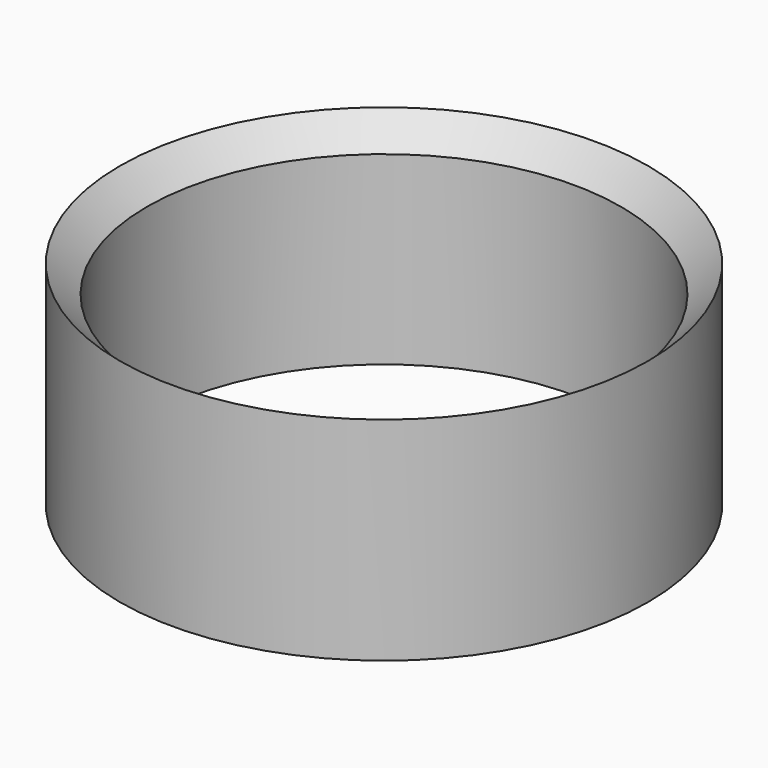
from build123d import *

# Parameters (mm, degrees)
F0_R     = 27.375
F0_R_2   = 24.565
F1_DEPTH = 22.09


# Not quite as in the source:
# - a fillet or chamfer that OpenCascade refuses, or shapes differently, is made with other operations: its cross-section is extruded or revolved along the edge and cut away or added


with BuildPart() as f1:
    # F0 (on Top) → F1 (new body)
    with BuildSketch(Plane.XY):
        Circle(F0_R)
        Circle(F0_R_2, mode=Mode.SUBTRACT)
    extrude(amount=F1_DEPTH)

    # F2: chamfer of 2.9 on 1 edges, made by hand

    # F2_s1 → F2_t2 (revolve, cut)
    with BuildSketch(Plane.XZ):
        Polygon((24.565, 19.19), (27.465, 22.09), (24.565, 22.09), align=None)
    revolve(axis=Axis((0, 0, 22.09), (0, 0, 1)), mode=Mode.SUBTRACT)


solid = f1.part
